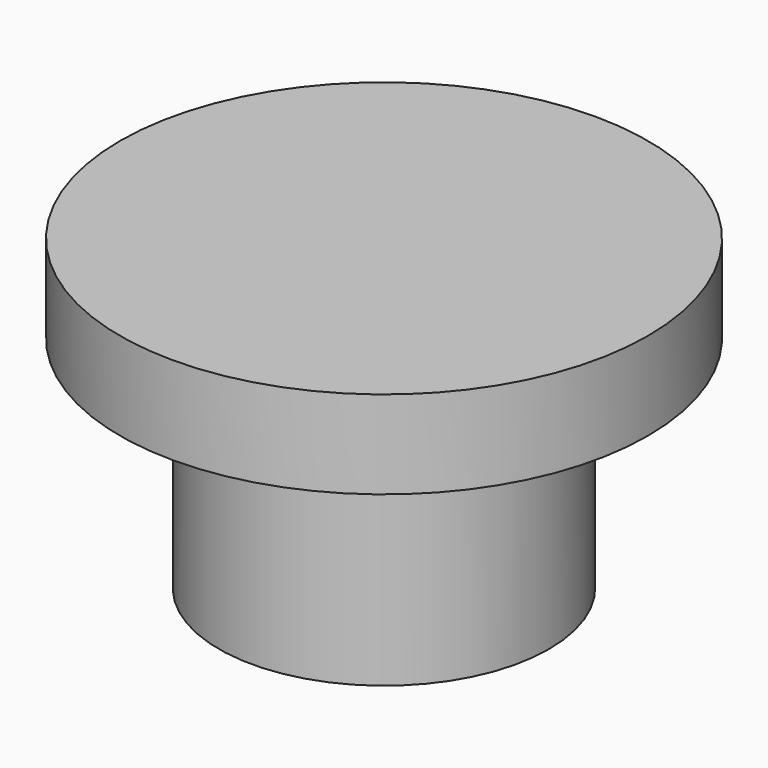
from build123d import *

# Parameters (mm, degrees)
F0_R     = 2.9765625
F1_DEPTH = 3.96875
F2_R     = 4.7625
F3_DEPTH = 1.5875


# Not quite as in the source:
# - a length typed as a fraction of an inch, garbled in the dataset ("3 / 203.2 mm" for 3/8 in), is restored


with BuildPart() as f1:
    # F0 (on Top) → F1 (new body)
    with BuildSketch(Plane.XY):
        Circle(F0_R)
    extrude(amount=F1_DEPTH)

    # F2 (on face) → F3 (join)
    with BuildSketch(Plane.XY.offset(3.96875)):
        Circle(F2_R)
    extrude(amount=F3_DEPTH)


solid = f1.part
